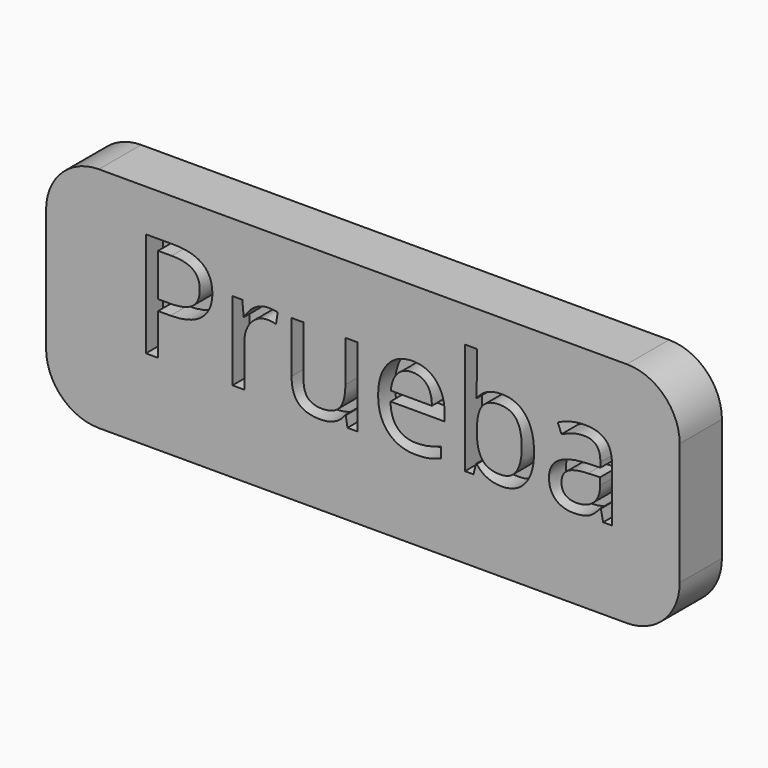
from build123d import *

# Parameters (mm, degrees)
F0_W         = 60
F0_H         = 21.5827333707
F1_DEPTH     = 5
F2_TEXT_SIZE = 13.9024761868
F3_DEPTH     = 2
F4_R         = 5


# Not quite as in the source:
# - Text() gives the source's letters only with a copy of the font that has no kerning and outlines rounded to 1/6400 em; it was checked with that copy


with BuildPart() as f1:
    # F0 (on Front) → F1 (new body)
    with BuildSketch(Plane.XZ):
        with Locations((-1.5303771943, 7.4605825357)):
            Rectangle(F0_W, F0_H)
    extrude(amount=F1_DEPTH)

    # F2 (on face) → F3 (cut)
    with BuildSketch(Plane.XZ.offset(5)):
        with Locations((-23.4436765313, 4.349435214)):
            Text('Prueba', F2_TEXT_SIZE, font='Open Sans', text_align=(TextAlign.LEFT, TextAlign.BOTTOM))
    extrude(amount=-F3_DEPTH, mode=Mode.SUBTRACT)

    # F4
    f4_edges = [f1.edges().sort_by_distance(p)[0] for p in [
        (28.469623, -2.5, 18.251949),
        (28.469623, -2.5, -3.330784),
        (-31.530377, -2.5, 18.251949),
        (-31.530377, -2.5, -3.330784),
    ]]
    fillet(f4_edges, radius=F4_R)


solid = f1.part
